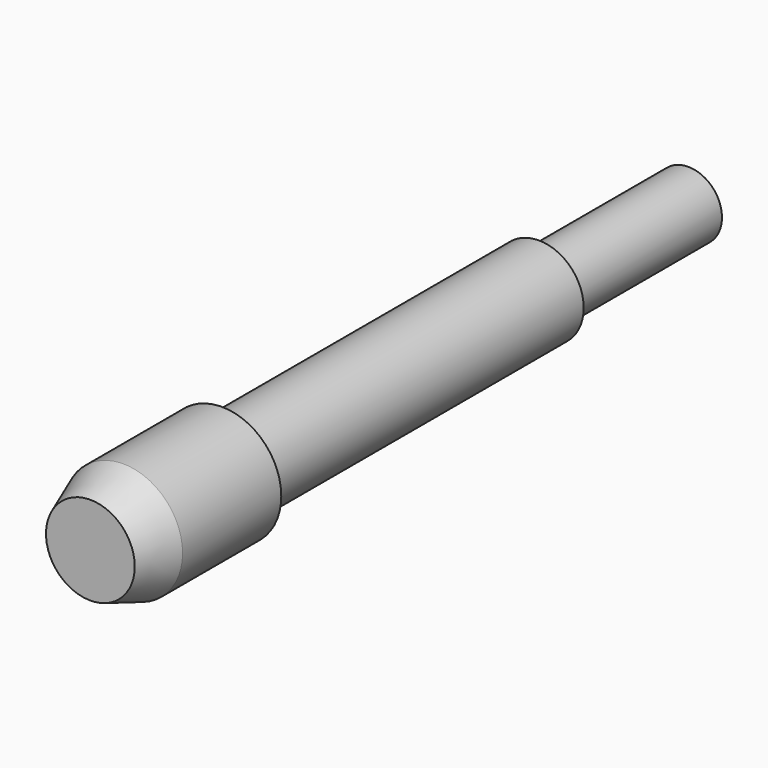
from build123d import *

# Parameters (mm, degrees)
F0_R     = 7.9375
F1_DEPTH = 22
F2_R     = 6
F3_DEPTH = 78
F4_R     = 6
F4_R_2   = 4.5
F5_DEPTH = 25
F6_SIZE2 = 5.4949548389
F6_SIZE  = 2


# Not quite as in the source:
# - a feature names something its author has since deleted; it is built from what else it names


with BuildPart() as f1:
    # F0 (on Front) → F1 (new body)
    with BuildSketch(Plane.XZ):
        Circle(F0_R)
    extrude(amount=F1_DEPTH)

    # F2 (on Front) → F3 (join)
    with BuildSketch(Plane.XZ):
        Circle(F2_R)
    extrude(amount=-F3_DEPTH)

    # F4 (on face) → F5 (cut)
    with BuildSketch(Plane(origin=(0, 78, 0), x_dir=(-1, 0, 0), z_dir=(0, 1, 0))):
        Circle(F4_R)
        Circle(F4_R_2, mode=Mode.SUBTRACT)
    extrude(amount=-F5_DEPTH, mode=Mode.SUBTRACT)

    # F6
    f6_edges = [f1.edges().sort_by_distance(p)[0] for p in [
        (-7.9375, -22, 0),
    ]]
    f6_side = f1.faces().sort_by_distance((0, -22, 0))[0]
    chamfer(f6_edges, length=F6_SIZE, length2=F6_SIZE2, reference=f6_side)


solid = f1.part
